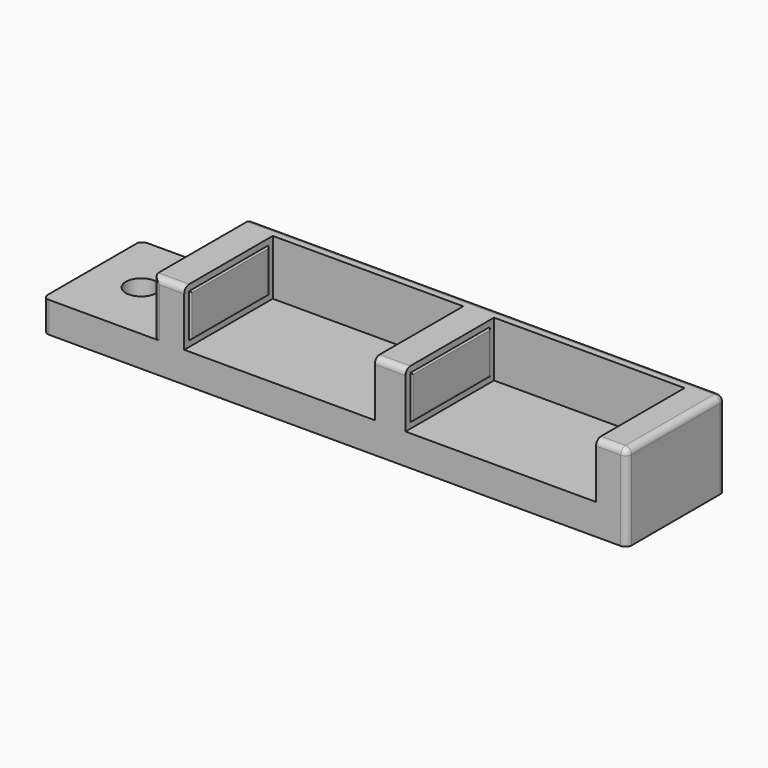
from build123d import *

# Parameters (mm, degrees)
F0_W      = 18
F0_H      = 20
F0_R      = 2.5
F0_W_2    = 31
F0_H_2    = 18
F0_H_3    = 2
F1_DEPTH  = 5
F2_DEPTH  = 14
F3_W      = 16
F3_H      = 7
F5_W      = 16
F5_H      = 7
F7_DEPTH  = 0.25
F4_W      = 16
F4_H      = 7
F6_W      = 16
F6_H      = 7
F8_DEPTH  = 0.25
F9_R      = 0.24999
F10_R     = 1
F11_W     = 20
F11_H     = 6
F12_DEPTH = 2
F13_SIZE  = 1


# Not quite as in the source:
# - a fillet or chamfer is up to 0.001 mm smaller than in the source, because OpenCascade refuses the exact size


with BuildPart() as f1:
    # F0 (on Top) → F1 (new body)
    with BuildSketch(Plane.XY):
        with Locations((-38.5, 0)):
            Rectangle(F0_W, F0_H)
        with Locations((-39.5, 0)):
            Circle(F0_R, mode=Mode.SUBTRACT)
        Polygon((-24.5, 10), (-29.5, 10), (-29.5, -10), (-24.5, -10), (-24.5, 8), align=None)
        with Locations((-9, -1)):
            Rectangle(F0_W_2, F0_H_2)
        Polygon((11.5, 10), (6.5, 10), (6.5, 8), (6.5, -10), (11.5, -10), (11.5, 8), align=None)
        Polygon((47.5, 10), (42.5, 10), (42.5, 8), (42.5, -10), (47.5, -10), align=None)
        with Locations((-9, 9)):
            Rectangle(F0_W_2, F0_H_3)
        with Locations((27, -1)):
            Rectangle(F0_W_2, F0_H_2)
        with Locations((27, 9)):
            Rectangle(F0_W_2, F0_H_3)
    extrude(amount=F1_DEPTH)

    # F0 (on Top) → F2 (join)
    with BuildSketch(Plane.XY):
        Polygon((-24.5, 10), (-29.5, 10), (-29.5, -10), (-24.5, -10), (-24.5, 8), align=None)
        Polygon((11.5, 10), (6.5, 10), (6.5, 8), (6.5, -10), (11.5, -10), (11.5, 8), align=None)
        Polygon((47.5, 10), (42.5, 10), (42.5, 8), (42.5, -10), (47.5, -10), align=None)
        with Locations((-9, 9)):
            Rectangle(F0_W_2, F0_H_3)
        with Locations((27, 9)):
            Rectangle(F0_W_2, F0_H_3)
    extrude(amount=F2_DEPTH)

    # F3 (on face) + F5 (on face) → F7 (join)
    with BuildSketch(Plane.YZ.offset(-24.5)):
        with Locations((-1, 9.5)):
            Rectangle(F3_W, F3_H)
    with BuildSketch(Plane.YZ.offset(11.5)):
        with Locations((-1, 9.5)):
            Rectangle(F5_W, F5_H)
    extrude(amount=F7_DEPTH)

    # F4 (on face) + F6 (on face) → F8 (join)
    with BuildSketch(Plane(origin=(6.5, 0, 0), x_dir=(0, -1, 0), z_dir=(-1, 0, 0))):
        with Locations((1, 9.5)):
            Rectangle(F4_W, F4_H)
    with BuildSketch(Plane(origin=(42.5, 0, 0), x_dir=(0, -1, 0), z_dir=(-1, 0, 0))):
        with Locations((1, 9.5)):
            Rectangle(F6_W, F6_H)
    extrude(amount=F8_DEPTH)

    # F9 (radius 0.25 in the source; OpenCascade refuses exactly that, so slightly less here)
    f9_edges = [f1.edges().sort_by_distance(p)[0] for p in [
        (-24.25, -1, 13),
        (-24.25, -9, 9.5),
        (-24.25, -1, 6),
        (-24.25, 7, 9.5),
        (6.25, 7, 9.5),
        (6.25, -1, 6),
        (6.25, -9, 9.5),
        (6.25, -1, 13),
        (11.75, -1, 13),
        (11.75, -9, 9.5),
        (11.75, -1, 6),
        (11.75, 7, 9.5),
        (42.25, -1, 13),
        (42.25, 7, 9.5),
        (42.25, -1, 6),
        (42.25, -9, 9.5),
    ]]
    fillet(f9_edges, radius=F9_R)

    # F10
    f10_edges = [f1.edges().sort_by_distance(p)[0] for p in [
        (-27, -10, 14),
        (9, -10, 14),
        (45, -10, 14),
        (9, 10, 14),
        (-47.5, -10, 2.5),
        (-47.5, 10, 2.5),
        (47.5, -10, 7),
        (47.5, 10, 7),
        (47.5, 0, 14),
        (-29.5, -10, 9.5),
        (-29.5, 10, 9.5),
    ]]
    fillet(f10_edges, radius=F10_R)

    # F11 (on face) → F12 (join)
    with BuildSketch(Plane.XY):
        with Locations((27.5, 0)):
            Rectangle(F11_W, F11_H)
    extrude(amount=-F12_DEPTH)

    # F13
    f13_edges = [f1.edges().sort_by_distance(p)[0] for p in [
        (27.5, -3, -2),
        (27.5, 3, -2),
    ]]
    chamfer(f13_edges, length=F13_SIZE)


solid = f1.part
